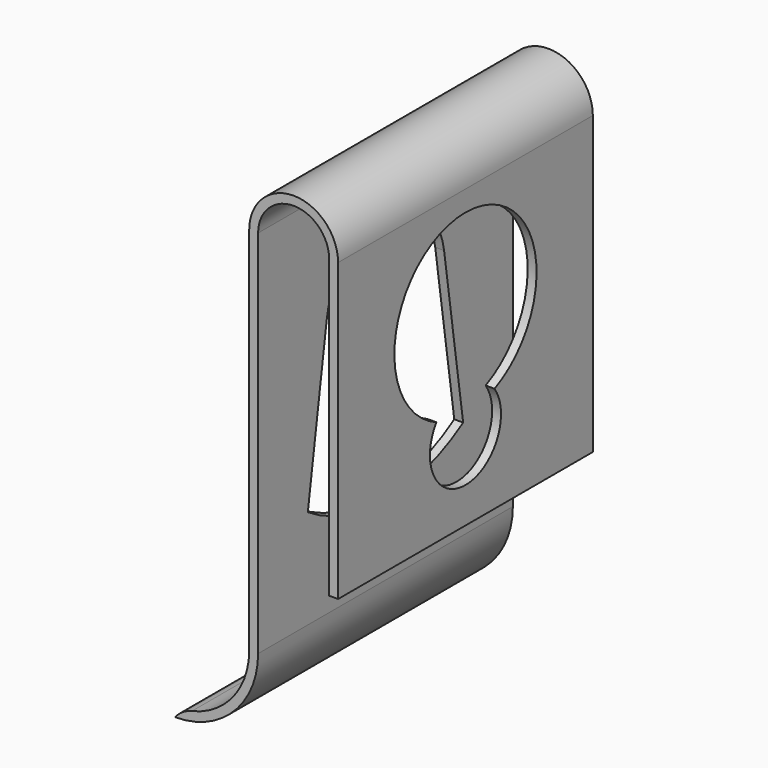
from build123d import *

# Parameters (mm, degrees)
F1_DEPTH    = 21.5
F3_DEPTH    = 1
F5_DEPTH    = 1
F6_T1_DEPTH = 27.2031140795


# Not quite as in the source:
# - a fillet or chamfer that OpenCascade refuses, or shapes differently, is made with other operations: its cross-section is extruded or revolved along the edge and cut away or added


with BuildPart() as f1:
    # F0 (on Front) → F1 (new body)
    with BuildSketch(Plane.XZ):
        with BuildLine():
            Line((-3, 0), (-3, -25))
            ThreePointArc((-3, -25), (-4.4644660941, -28.5355339059), (-8, -30))
            Line((-8, -30), (-8, -30.6))
            ThreePointArc((-8, -30.6), (-4.0402020254, -28.9597979746), (-2.4, -25))
            Line((-2.4, -25), (-2.4, 0))
            ThreePointArc((-2.4, 0), (0, 2.4), (2.4, 0))
            Line((2.4, 0), (2.4, -20))
            Line((2.4, -20), (3, -20))
            Line((3, -20), (3, 0))
            ThreePointArc((3, 0), (0, 3), (-3, 0))
        make_face()
    extrude(amount=F1_DEPTH)

    # F2 (on face) → F3 (cut)
    with BuildSketch(Plane(origin=(-3, 0, 0), x_dir=(0, -1, 0), z_dir=(-1, 0, 0))):
        with BuildLine():
            Line((5.8037092493, -7.4218333804), (4.195739785, -18.3036730319))
            ThreePointArc((4.195739785, -18.3036730319), (10.75, -20.2517243137), (17.304260215, -18.3036730319))
            Line((17.304260215, -18.3036730319), (15.6962907507, -7.4218333804))
            ThreePointArc((15.6962907507, -7.4218333804), (10.75, -3.1527285914), (5.8037092493, -7.4218333804))
        make_face()
    extrude(amount=-F3_DEPTH, mode=Mode.SUBTRACT)

    # F4 (on face) → F5 (cut)
    with BuildSketch(Plane.YZ.offset(3)):
        with BuildLine():
            ThreePointArc((-13.2016747035, -12.8677467976), (-10.75, -17.5967034623), (-8.2983252965, -12.8677467976))
            ThreePointArc((-8.2983252965, -12.8677467976), (-10.75, -1.3914988898), (-13.2016747035, -12.8677467976))
        make_face()
    extrude(amount=-F5_DEPTH, mode=Mode.SUBTRACT)

    # F6: fillet of radius 2 on 1 edges, made by hand

    # F6_s2 → F6_t1 (cut)
    with BuildSketch(Plane.XZ.offset(-2.8515570398)):
        with BuildLine():
            ThreePointArc((-8, -30.6), (-7.4967757486, -30.136601148), (-6.8668213437, -29.8698979592))
            ThreePointArc((-6.8668213437, -29.8698979592), (-7.429688592, -29.9673680051), (-8, -30))
            Line((-8, -30), (-8, -30.6))
        make_face()
    extrude(amount=F6_T1_DEPTH, mode=Mode.SUBTRACT)


solid = f1.part
